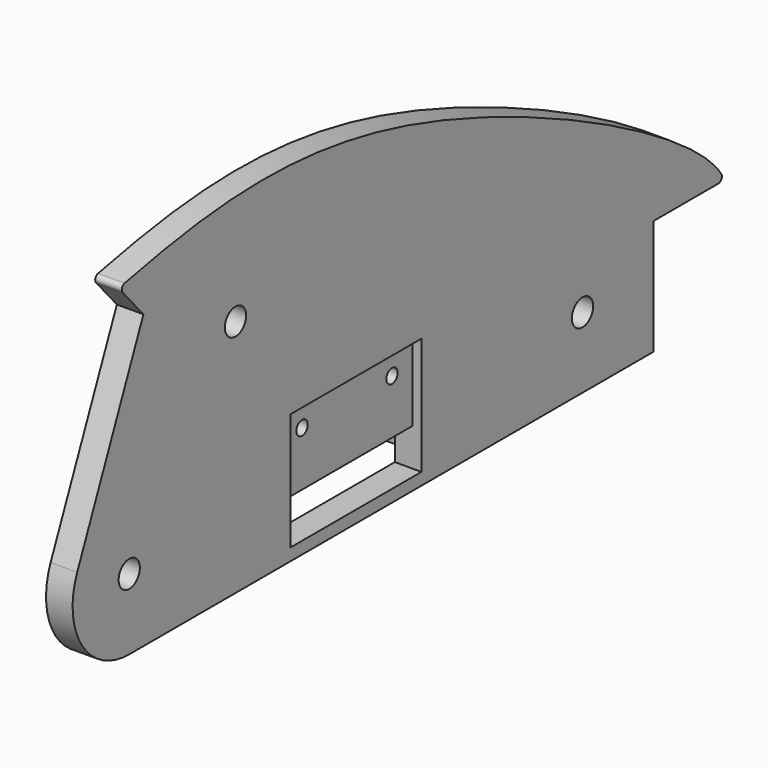
from build123d import *

# Parameters (mm, degrees)
F0_R      = 1.5
F1_DEPTH  = 3
F2_W      = 18.5
F2_H      = 6.625
F3_DEPTH  = 25
F4_W      = 18.5
F4_H      = 9
F5_DEPTH  = 1
F6_DEPTH  = 2
F8_D      = 1.6
F9_SIZE   = 0.99999
F10_W     = 6
F10_H     = 6
F11_DEPTH = 8
F12_R     = 2.99999
F13_W     = 6
F13_H     = 6
F14_DEPTH = 8
F15_R     = 2.99999
F17_D     = 2.5
F18_R     = 0.5
F19_DEPTH = 9.625


# Not quite as in the source:
# - a fillet or chamfer is up to 0.001 mm smaller than in the source, because OpenCascade refuses the exact size


with BuildPart() as f1:
    # F0 (on Right) → F1 (new body)
    with BuildSketch(Plane.YZ):
        with BuildLine():
            Line((-64, -8), (10, -8))
            Line((10, -8), (10, 5))
            Line((10, 5), (20, 5))
            add(Edge.make_bspline(
                [(-65.5, 29), (-53.1884357333, 31.5765216947), (-28.2810822655, 35.0271902112), (17.668255518, 10.972023372), (20, 5)],
                knots=[0, 0, 0, 0, 0.471377868, 1, 1, 1, 1], degree=3))
            Line((-65.5, 29), (-62, 25))
            Line((-62, 25), (-71.3544447211, 3.1483555777))
            ThreePointArc((-71.3544447211, 3.1483555777), (-70.677830659, -4.4052897395), (-64, -8))
        make_face()
        with Locations((-64, 0)):
            Circle(F0_R, mode=Mode.SUBTRACT)
        Circle(F0_R, mode=Mode.SUBTRACT)
        with Locations((-49, 19)):
            Circle(F0_R, mode=Mode.SUBTRACT)
    extrude(amount=F1_DEPTH)

    # F2 (on face) → F3 (cut)
    with BuildSketch(Plane.YZ.offset(3)):
        with Locations((-32, 3.3125)):
            Rectangle(F2_W, F2_H)
        with Locations((-32, -3.3125)):
            Rectangle(F2_W, F2_H)
    extrude(amount=-F3_DEPTH, mode=Mode.SUBTRACT)

    # F4 (on face) → F5 (join)
    with BuildSketch(Plane(origin=(0, 0, 0), x_dir=(0, -1, 0), z_dir=(-1, 0, 0))):
        with Locations((32, 2.125)):
            Rectangle(F4_W, F4_H)
        Polygon((42.25, -2.375), (42.25, 7.625), (21.75, 7.625), (21.75, -2.375), (22.75, -2.375), (22.75, 6.625), (41.25, 6.625), (41.25, -2.375), align=None)
    extrude(amount=F5_DEPTH)

    # F6 (add): a face of the model
    f6_faces = [f1.faces().sort_by_distance(p)[0] for p in [
        (0, -32, 2.125),
    ]]
    extrude(f6_faces, amount=F6_DEPTH)

    # F8 (through all)
    with Locations(Plane.YZ.offset(2)):
        with Locations((-38.35, 3.775), (-25.65, 3.775)):
            Hole(F8_D / 2)

    # F9 (size 1 in the source; OpenCascade refuses exactly that, so slightly less here)
    f9_edges = [f1.edges().sort_by_distance(p)[0] for p in [
        (-1, -21.75, 2.625),
        (-1, -42.25, 2.625),
    ]]
    chamfer(f9_edges, length=F9_SIZE)

    # F10 (on face) → F11 (join)
    with BuildSketch(Plane(origin=(0, 0, 0), x_dir=(0, -1, 0), z_dir=(-1, 0, 0))):
        with Locations((49, 4.625)):
            Rectangle(F10_W, F10_H)
    extrude(amount=F11_DEPTH)

    # F12 (radius 3 in the source; OpenCascade refuses exactly that, so slightly less here)
    f12_edges = [f1.edges().sort_by_distance(p)[0] for p in [
        (-8, -52, 4.625),
        (-8, -46, 4.625),
    ]]
    fillet(f12_edges, radius=F12_R)

    # F13 (on face) → F14 (join)
    with BuildSketch(Plane(origin=(0, 0, 0), x_dir=(0, -1, 0), z_dir=(-1, 0, 0))):
        with Locations((15, 4.625)):
            Rectangle(F13_W, F13_H)
    extrude(amount=F14_DEPTH)

    # F15 (radius 3 in the source; OpenCascade refuses exactly that, so slightly less here)
    f15_edges = [f1.edges().sort_by_distance(p)[0] for p in [
        (-8, -12, 4.625),
        (-8, -18, 4.625),
    ]]
    fillet(f15_edges, radius=F15_R)

    # F17 (through all)
    with Locations(Plane.XY.offset(7.625)):
        with Locations((-5, -49), (-5, -15)):
            Hole(F17_D / 2)

    # F18
    f18_edges = [f1.edges().sort_by_distance(p)[0] for p in [
        (1.5, -65.5, 29),
        (1.5, 20, 5),
    ]]
    fillet(f18_edges, radius=F18_R)

    # F19 (add): faces of the model
    f19_faces = [f1.faces().sort_by_distance(p)[0] for p in [
        (-3.5469743881, -15, 1.625),
        (-3.5469743881, -49, 1.625),
    ]]
    extrude(f19_faces, amount=F19_DEPTH)


solid = f1.part
